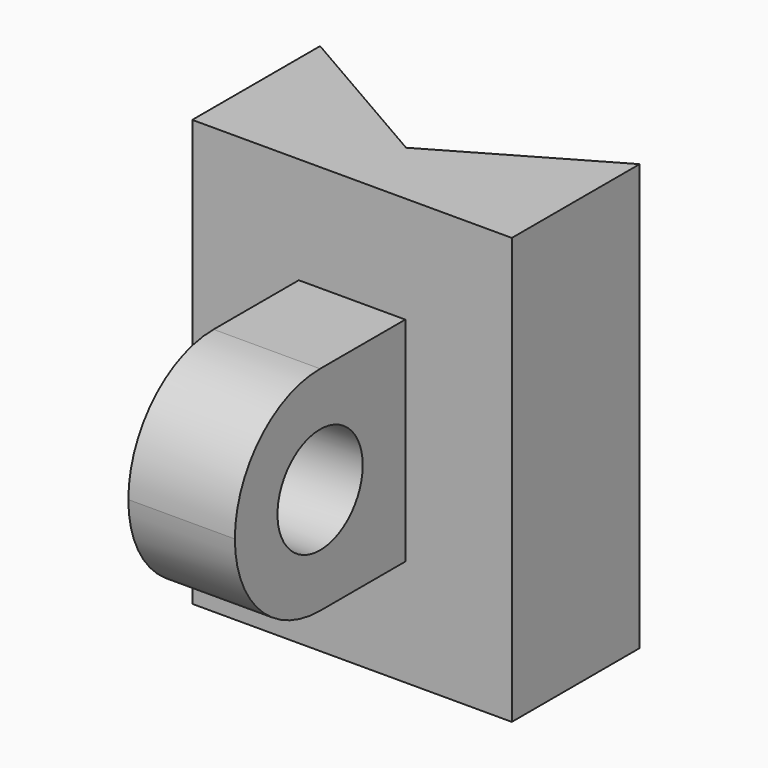
from build123d import *

# Parameters (mm, degrees)
F0_W     = 30
F0_H     = 40
F1_DEPTH = 15
F2_W     = 10
F2_H     = 20
F3_DEPTH = 20
F4_R     = 5
F5_DEPTH = 20.001
F6_R     = 9.99999
F8_DEPTH = 40.001


# Not quite as in the source:
# - a fillet or chamfer is up to 0.001 mm smaller than in the source, because OpenCascade refuses the exact size


with BuildPart() as f1:
    # F0 (on Front) → F1 (new body)
    with BuildSketch(Plane.XZ):
        Rectangle(F0_W, F0_H)
    extrude(amount=F1_DEPTH)

    # F2 (on face) → F3 (join)
    with BuildSketch(Plane.XZ.offset(15)):
        Rectangle(F2_W, F2_H)
    extrude(amount=F3_DEPTH)

    # F4 (on face) → F5 (cut, through all)
    with BuildSketch(Plane.YZ.offset(5)):
        with Locations((-25, 0)):
            Circle(F4_R)
    extrude(amount=-F5_DEPTH, mode=Mode.SUBTRACT)

    # F6 (radius 10 in the source; OpenCascade refuses exactly that, so slightly less here)
    f6_edges = [f1.edges().sort_by_distance(p)[0] for p in [
        (0, -35, 10),
        (0, -35, -10),
    ]]
    fillet(f6_edges, radius=F6_R)

    # F7 (on face) → F8 (cut, through all)
    with BuildSketch(Plane.XY.offset(20)):
        Polygon((15, 0), (-15, 0), (0, -8.6602540378), align=None)
    extrude(amount=-F8_DEPTH, mode=Mode.SUBTRACT)


solid = f1.part
